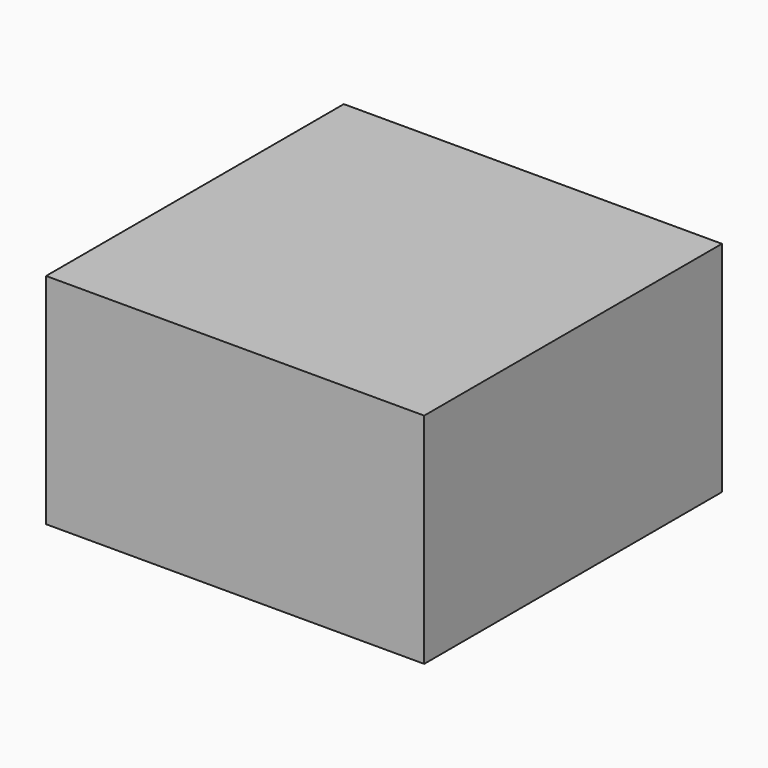
from build123d import *

# Parameters (mm, degrees)
F0_W     = 69.8630958796
F0_H     = 137.5265717506
F2_DEPTH = 80.772


# Not quite as in the source:
# - the program builds the solid bodies; features that only make, move or delete a surface that nothing else refers to are left out


with BuildPart() as f2:
    # F0 (on Top) → F2 (new body)
    with BuildSketch(Plane.XY):
        with Locations((-34.9315479398, 0)):
            Rectangle(F0_W, F0_H)
        with Locations((34.9315479398, 0)):
            Rectangle(F0_W, F0_H)
    extrude(amount=-F2_DEPTH)


solid = f2.part
